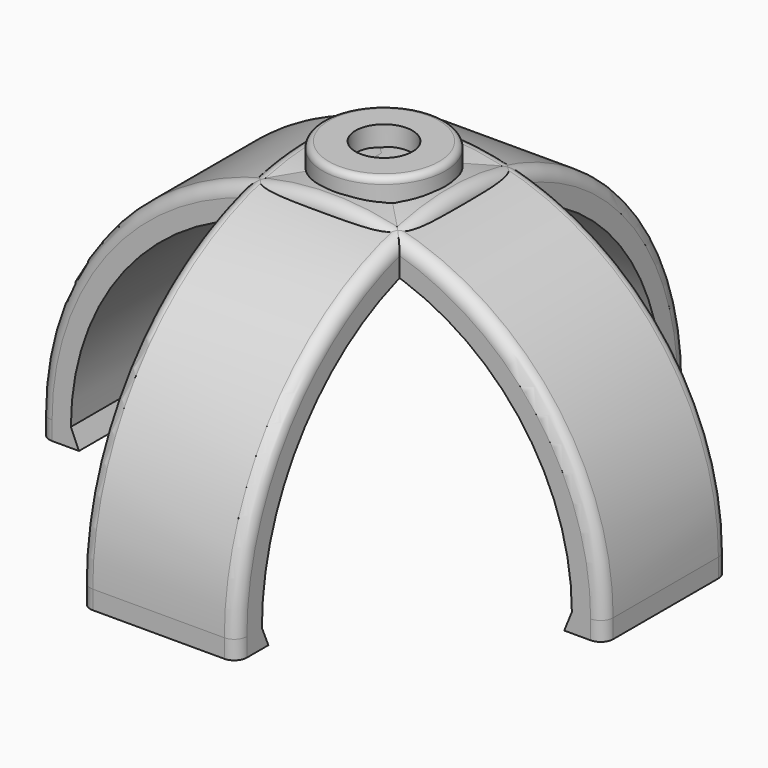
from build123d import *

# Parameters (mm, degrees)
F1_DEPTH = 12.5
F4_ANGLE = 90
F5_R     = 2
F5_2_R   = 2
F6_R     = 9.811106596
F6_R_2   = 4.5458259895
F7_DEPTH = 5
F8_R     = 1


with BuildPart() as f1:
    # F0 (on Front) → F1 (new body, symmetric)
    with BuildSketch(Plane.XZ):
        with BuildLine():
            ThreePointArc((-40, 0), (0, 40), (40, 0))
            Line((40, 0), (38.7801602483, -3.0118847469))
            Line((38.7801602483, -3.0118847469), (45, -3.0118847469))
            Line((45, -3.0118847469), (45, 0))
            ThreePointArc((45, 0), (0, 45), (-45, 0))
            Line((-45, 0), (-45, -2.9643927701))
            Line((-45, -2.9643927701), (-38.7012884021, -2.9643927701))
            Line((-38.7012884021, -2.9643927701), (-40, 0))
        make_face()
    extrude(amount=F1_DEPTH, both=True)


with BuildPart() as f4_1:
    # F4: copy of F1
    add(f1.part.rotate(Axis((0, 0, 43.1), (0, 0, 1)), F4_ANGLE))

    # F5#2
    f5_2_edges = [f4_1.edges().sort_by_distance(p)[0] for p in [
        (0, 45, 0),
        (-12.5, 0, 45),
        (0, -45, 0),
        (12.5, 0, 45),
        (-12.5, -45, -1.482196),
        (12.5, -45, -1.482196),
        (-12.5, 45, -1.505942),
        (12.5, 45, -1.505942),
    ]]
    fillet(f5_2_edges, radius=F5_2_R)


with BuildPart() as f1_1:
    add(f1.part)

    # F5
    f5_edges = [f1_1.edges().sort_by_distance(p)[0] for p in [
        (0, -12.5, 45),
        (0, 12.5, 45),
        (-45, 12.5, -1.482196),
        (-45, -12.5, -1.482196),
        (45, 12.5, -1.505942),
        (45, -12.5, -1.505942),
    ]]
    fillet(f5_edges, radius=F5_R)


with BuildPart() as f7:
    # F6 (on offset) → F7 (new body)
    with BuildSketch(Plane.XY.offset(43.1)):
        Circle(F6_R)
        Circle(F6_R_2, mode=Mode.SUBTRACT)
    extrude(amount=F7_DEPTH)

    # F8
    f8_edges = [f7.edges().sort_by_distance(p)[0] for p in [
        (9.811107, 0, 45.6),
        (-9.811107, 0, 43.1),
        (-9.811107, 0, 48.1),
    ]]
    fillet(f8_edges, radius=F8_R)


solid = Compound([f4_1.part, f1_1.part, f7.part])
